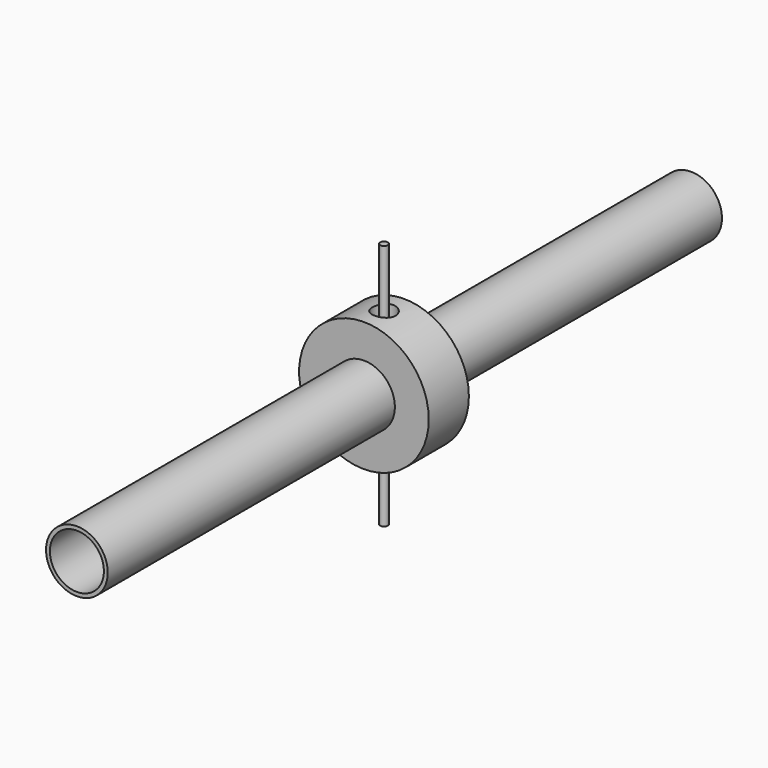
from build123d import *

# Parameters (mm, degrees)
F0_R      = 53.34
F0_R_2    = 22.225
F1_DEPTH  = 20.6375
F6_DEPTH  = 20.6375
F5_R      = 9.525
F5_R_2    = 3.302
F7_DEPTH  = 19.05
F8_DEPTH  = 32.3616602869
F4_R      = 9.525
F4_R_2    = 3.302
F9_DEPTH  = 19.05
F10_DEPTH = 32.3616602869
F13_W     = 2.032
F13_H     = 3.556
F15_R     = 3.175
F16_DEPTH = 101.6
F19_R     = 25.4
F19_R_2   = 22.225
F20_DEPTH = 304.8
F21_R     = 25.4
F21_R_2   = 22.225
F22_DEPTH = 304.8


# Not quite as in the source:
# - the program builds the solid bodies; features that only make, move or delete a surface that nothing else refers to are left out


with BuildPart() as f1:
    # F0 (on Front) → F1 (new body)
    with BuildSketch(Plane.XZ):
        Circle(F0_R)
        Circle(F0_R_2, mode=Mode.SUBTRACT)
    extrude(amount=-F1_DEPTH)

    # F0 (on Front) → F6 (join)
    with BuildSketch(Plane.XZ):
        Circle(F0_R)
        Circle(F0_R_2, mode=Mode.SUBTRACT)
    extrude(amount=F6_DEPTH)

    # F5 (on offset) → F7 (cut)
    with BuildSketch(Plane.XY.offset(-53.34)):
        Circle(F5_R)
        Circle(F5_R_2, mode=Mode.SUBTRACT)
        Circle(F5_R_2)
    extrude(amount=F7_DEPTH, mode=Mode.SUBTRACT)

    # F5 (on offset) → F8 (cut, up to face)
    with BuildSketch(Plane.XY.offset(-53.34)):
        Circle(F5_R_2)
    extrude(amount=F8_DEPTH, mode=Mode.SUBTRACT)

    # F4 (on offset) → F9 (cut)
    with BuildSketch(Plane.XY.offset(53.34)):
        Circle(F4_R)
        Circle(F4_R_2, mode=Mode.SUBTRACT)
        Circle(F4_R_2)
    extrude(amount=-F9_DEPTH, mode=Mode.SUBTRACT)

    # F4 (on offset) → F10 (cut, up to face)
    with BuildSketch(Plane.XY.offset(53.34)):
        Circle(F4_R_2)
    extrude(amount=-F10_DEPTH, mode=Mode.SUBTRACT)

    # F11 (on Right) → F12 (revolve, cut)
    with BuildSketch(Plane.YZ):
        Polygon((6.35, 34.29), (3.302, 34.29), (3.302, 29.21), align=None)
        Polygon((3.302, -29.21), (3.302, -34.29), (6.35, -34.29), align=None)
    revolve(axis=Axis((0, 0, 6.9711627439), (0, 0, 1)), mode=Mode.SUBTRACT)

    # F13 (on Top) → F14 (revolve, cut)
    with BuildSketch(Plane.XY):
        Polygon((-25.4254, 11.1125), (-22.225, 11.1125), (-22.225, 20.6375), (-25.4254, 20.6375), (-25.4254, 17.653), (-25.4254, 14.097), align=None)
        Polygon((-22.225, -20.6375), (-22.225, -11.1125), (-25.4254, -11.1125), (-25.4254, -14.097), (-25.4254, -17.653), (-25.4254, -20.6375), align=None)
        with Locations((-26.4414, 15.875)):
            Rectangle(F13_W, F13_H)
        with Locations((-26.4414, -15.875)):
            Rectangle(F13_W, F13_H)
    revolve(axis=Axis((0, 5.55625, 0), (0, 1, 0)), mode=Mode.SUBTRACT)


with BuildPart() as f16:
    # F15 (on Top) → F16 (new body, symmetric)
    with BuildSketch(Plane.XY):
        Circle(F15_R)
    extrude(amount=F16_DEPTH, both=True)


with BuildPart() as f20:
    # F19 (on face) → F20 (new body)
    with BuildSketch(Plane.XZ.offset(11.1125)):
        Circle(F19_R)
        Circle(F19_R_2, mode=Mode.SUBTRACT)
    extrude(amount=F20_DEPTH)


with BuildPart() as f22:
    # F21 (on face) → F22 (new body)
    with BuildSketch(Plane(origin=(0, 11.1125, 0), x_dir=(-1, 0, 0), z_dir=(0, 1, 0))):
        Circle(F21_R)
        Circle(F21_R_2, mode=Mode.SUBTRACT)
    extrude(amount=F22_DEPTH)


solid = Compound([f1.part, f16.part, f20.part, f22.part])
